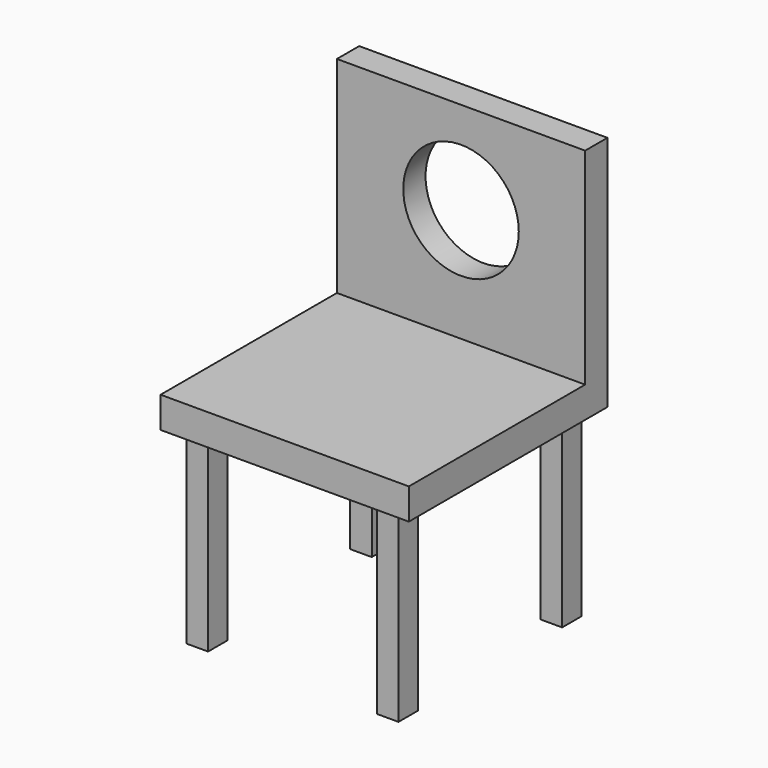
from build123d import *

# Parameters (mm, degrees)
F0_W     = 3.4663490951
F0_H     = 3.8823140785
F0_H_2   = 2.9117353261
F0_H_3   = 0.9705787525
F1_DEPTH = 5
F2_DEPTH = 30
F3_DEPTH = 38.19281
F4_R     = 9.3059115505
F5_DEPTH = 4.488162903


with BuildPart() as f1:
    # F0 (on Top) → F1 (new body)
    with BuildSketch(Plane.XY):
        Polygon((20, -20), (20, 15.512837097), (17.0732010156, 15.512837097), (17.0732010156, 14.5422583446), (13.6068519205, 14.5422583446), (13.6068519205, 15.512837097), (-13.6068519205, 15.512837097), (-13.6068519205, 14.5422583446), (-17.0732010156, 14.5422583446), (-17.0732010156, 15.512837097), (-20, 15.512837097), (-20, -20), align=None)
        with Locations((-15.340026468, -16.4834153838)):
            Rectangle(F0_W, F0_H, mode=Mode.SUBTRACT)
        with Locations((15.340026468, -16.4834153838)):
            Rectangle(F0_W, F0_H, mode=Mode.SUBTRACT)
        Polygon((20, 15.512837097), (20, 20), (-20, 20), (-20, 15.512837097), (-17.0732010156, 15.512837097), (-17.0732010156, 18.4245724231), (-13.6068519205, 18.4245724231), (-13.6068519205, 15.512837097), (13.6068519205, 15.512837097), (13.6068519205, 18.4245724231), (17.0732010156, 18.4245724231), (17.0732010156, 15.512837097), align=None)
        with Locations((15.340026468, -16.4834153838)):
            Rectangle(F0_W, F0_H)
        with Locations((-15.340026468, -16.4834153838)):
            Rectangle(F0_W, F0_H)
        with Locations((15.340026468, 16.9687047601)):
            Rectangle(F0_W, F0_H_2)
        with Locations((-15.340026468, 16.9687047601)):
            Rectangle(F0_W, F0_H_2)
        with Locations((15.340026468, 15.0275477208)):
            Rectangle(F0_W, F0_H_3)
        with Locations((-15.340026468, 15.0275477208)):
            Rectangle(F0_W, F0_H_3)
    extrude(amount=F1_DEPTH)

    # F0 (on Top) → F2 (join)
    with BuildSketch(Plane.XY):
        with Locations((15.340026468, -16.4834153838)):
            Rectangle(F0_W, F0_H)
        with Locations((-15.340026468, -16.4834153838)):
            Rectangle(F0_W, F0_H)
        with Locations((-15.340026468, 16.9687047601)):
            Rectangle(F0_W, F0_H_2)
        with Locations((15.340026468, 16.9687047601)):
            Rectangle(F0_W, F0_H_2)
        with Locations((15.340026468, 15.0275477208)):
            Rectangle(F0_W, F0_H_3)
        with Locations((-15.340026468, 15.0275477208)):
            Rectangle(F0_W, F0_H_3)
    extrude(amount=-F2_DEPTH)

    # F0 (on Top) → F3 (join)
    with BuildSketch(Plane.XY):
        Polygon((20, 15.512837097), (20, 20), (-20, 20), (-20, 15.512837097), (-17.0732010156, 15.512837097), (-17.0732010156, 18.4245724231), (-13.6068519205, 18.4245724231), (-13.6068519205, 15.512837097), (13.6068519205, 15.512837097), (13.6068519205, 18.4245724231), (17.0732010156, 18.4245724231), (17.0732010156, 15.512837097), align=None)
        with Locations((-15.340026468, 16.9687047601)):
            Rectangle(F0_W, F0_H_2)
        with Locations((15.340026468, 16.9687047601)):
            Rectangle(F0_W, F0_H_2)
    extrude(amount=F3_DEPTH)

    # F4 (on face) → F5 (cut, through all)
    with BuildSketch(Plane.XZ.offset(-15.512837097)):
        with Locations((0, 23.2225228101)):
            Circle(F4_R)
    extrude(amount=-F5_DEPTH, mode=Mode.SUBTRACT)


solid = f1.part
